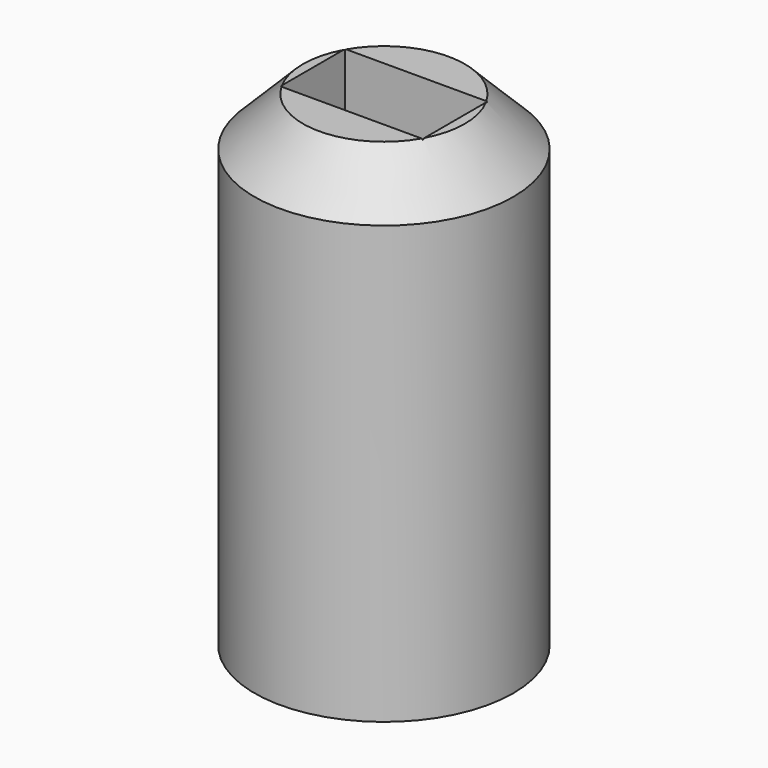
from build123d import *

# Parameters (mm, degrees)
F0_R     = 4
F0_R_2   = 2.6
F1_DEPTH = 15
F2_START = 6
F0_W     = 4.4
F0_H     = 2.5
F2_DEPTH = 9
F3_START = 6
F3_DEPTH = 6


# Not quite as in the source:
# - a fillet or chamfer that OpenCascade refuses, or shapes differently, is made with other operations: its cross-section is extruded or revolved along the edge and cut away or added


with BuildPart() as f1:
    # F0 (on Top) → F1 (new body)
    with BuildSketch(Plane.XY):
        Circle(F0_R)
        Circle(F0_R_2, mode=Mode.SUBTRACT)
    extrude(amount=F1_DEPTH)

    # F0 (on Top) → F2 (join)
    with BuildSketch(Plane.XY.offset(F2_START)):
        Circle(F0_R_2)
        Rectangle(F0_W, F0_H, mode=Mode.SUBTRACT)
    extrude(amount=F2_DEPTH)

    # F0 (on Top) → F3 (join)
    with BuildSketch(Plane.XY.offset(F3_START)):
        Rectangle(F0_W, F0_H)
    extrude(amount=F3_DEPTH)

    # F4: chamfer of 1.5 on 1 edges, made by hand

    # F4_s1 → F4_t2 (revolve, cut)
    with BuildSketch(Plane.XZ):
        Polygon((4, 13.5), (2.5, 15), (4, 15), align=None)
    revolve(axis=Axis((0, 0, 15), (0, 0, 1)), mode=Mode.SUBTRACT)


solid = f1.part
